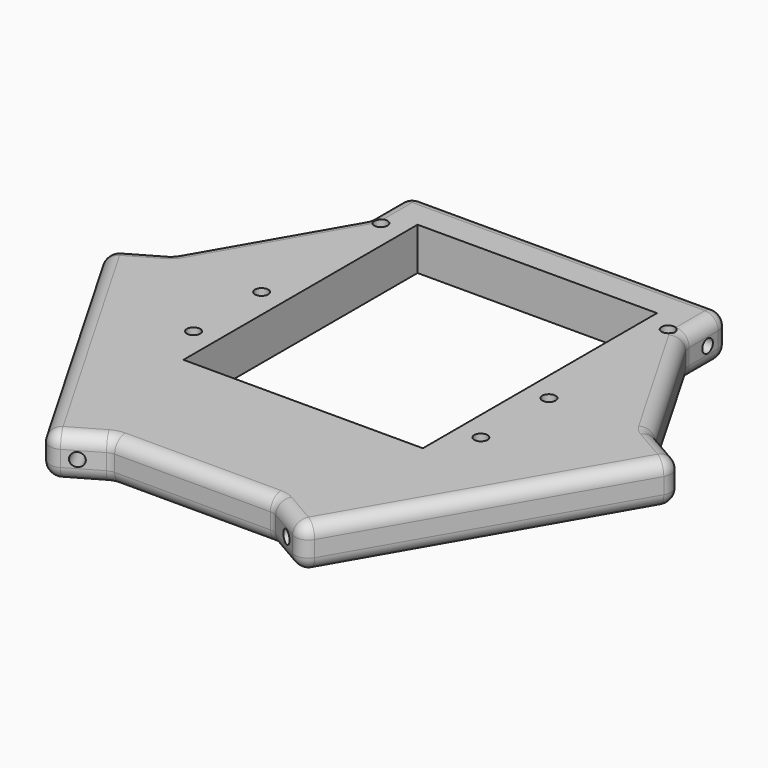
from build123d import *

# Parameters (mm, degrees)
F1_DEPTH = 8
F3_D     = 2.5
F5_D     = 2.5
F7_D     = 2.5
F8_F1_R  = 2.5
F8_F2_R  = 2.5
F9_D     = 2.5


with BuildPart() as f1:
    # F0 (on Top) → F1 (new body)
    with BuildSketch(Plane.XY):
        Polygon((-22.5, 35), (-30, 35), (-45.3108891325, 8.4807621135), (-15.3108891325, -43.4807621135), (15.3108891325, -43.4807621135), (45.3108891325, 8.4807621135), (30, 35), (22.5, 35), (22.5, 17.5), (22.5, -17.5), (-22.5, -17.5), (-22.5, 17.5), align=None)
        Polygon((-15.3108891325, -43.4807621135), (-45.3108891325, 8.4807621135), (-53.9711431703, 3.4807621135), (-23.9711431703, -48.4807621135), align=None)
        Polygon((30, 45), (-30, 45), (-30, 35), (-22.5, 35), (-22.5, 37.5), (22.5, 37.5), (22.5, 35), (30, 35), align=None)
        Polygon((53.9711431703, 3.4807621135), (45.3108891325, 8.4807621135), (15.3108891325, -43.4807621135), (23.9711431703, -48.4807621135), align=None)
    extrude(amount=F1_DEPTH)

    # F3 (through all)
    with Locations(Plane(origin=(-30, 0, 0), x_dir=(0, -1, 0), z_dir=(-1, 0, 0))):
        with Locations((-40, 4)):
            Hole(F3_D / 2)

    # F5 (through all)
    with Locations(Plane(origin=(15, -25.9807621135, 0), x_dir=(0.8660254038, 0.5, 0), z_dir=(0.5, -0.8660254038, 0))):
        with Locations((-40, 4)):
            Hole(F5_D / 2)

    # F7 (through all)
    with Locations(Plane(origin=(15, 25.9807621135, 0), x_dir=(-0.8660254038, 0.5, 0), z_dir=(0.5, 0.8660254038, 0))):
        with Locations((-40, 4)):
            Hole(F7_D / 2)

    # F8: fillet of radius 2.5 on 32 edges, made by hand

    # F8_f1
    f8_f1_edges = [f1.edges().sort_by_distance(p)[0] for p in [
        (-45.3108891325, 8.4807621135, 4),
        (-30, 35, 4),
        (30, 35, 4),
        (45.3108891325, 8.4807621135, 4),
        (15.3108891325, -43.4807621135, 4),
        (-15.3108891325, -43.4807621135, 4),
    ]]
    fillet(f8_f1_edges, radius=F8_F1_R)

    # F8_f2
    f8_f2_edges = [f1.edges().sort_by_distance(p)[0] for p in [
        (-37.6554445662, 21.7403810568, 8),
        (-30, 40.3349364905, 8),
        (0, 45, 8),
        (37.6554445662, 21.7403810568, 8),
        (30, 40.3349364905, 8),
        (49.9310796608, 5.8132938683, 8),
        (38.9711431703, -22.5, 8),
        (19.9310796608, -46.1482303588, 8),
        (0, -43.4807621135, 8),
        (-19.9310796608, -46.1482303588, 8),
        (-38.9711431703, -22.5, 8),
        (-49.9310796608, 5.8132938683, 8),
        (-53.9711431703, 3.4807621135, 4),
        (-30, 45, 4),
        (30, 45, 4),
        (53.9711431703, 3.4807621135, 4),
        (23.9711431703, -48.4807621135, 4),
        (-23.9711431703, -48.4807621135, 4),
        (-38.9711431703, -22.5, 0),
        (-37.6554445662, 21.7403810568, 0),
        (0, 45, 0),
        (30, 40.3349364905, 0),
        (38.9711431703, -22.5, 0),
        (19.9310796608, -46.1482303588, 0),
        (0, -43.4807621135, 0),
        (-19.9310796608, -46.1482303588, 0),
        (-15.2880637641, -43.5659475478, 0),
        (15.2880637641, -43.5659475478, 0),
        (30.0851854343, 35.0228253683, 0),
        (-30.0851854343, 35.0228253683, 0),
        (-45.3732491984, 8.5431221795, 0),
        (-45.3732491984, 8.5431221795, 8),
        (-15.2880637641, -43.5659475478, 8),
        (15.2880637641, -43.5659475478, 8),
        (45.3732491984, 8.5431221795, 8),
        (30.0851854343, 35.0228253683, 8),
        (-30.0851854343, 35.0228253683, 8),
    ]]
    fillet(f8_f2_edges, radius=F8_F2_R)

    # F9 (through all)
    with Locations(Plane(origin=(0, 0, 0), x_dir=(1, 0, 0), z_dir=(0, 0, -1))):
        with Locations((-27, -6.5), (-27, 9.5), (27, 9.5), (27, -6.5), (-27, -34.5), (27, -34.5)):
            Hole(F9_D / 2)


solid = f1.part
